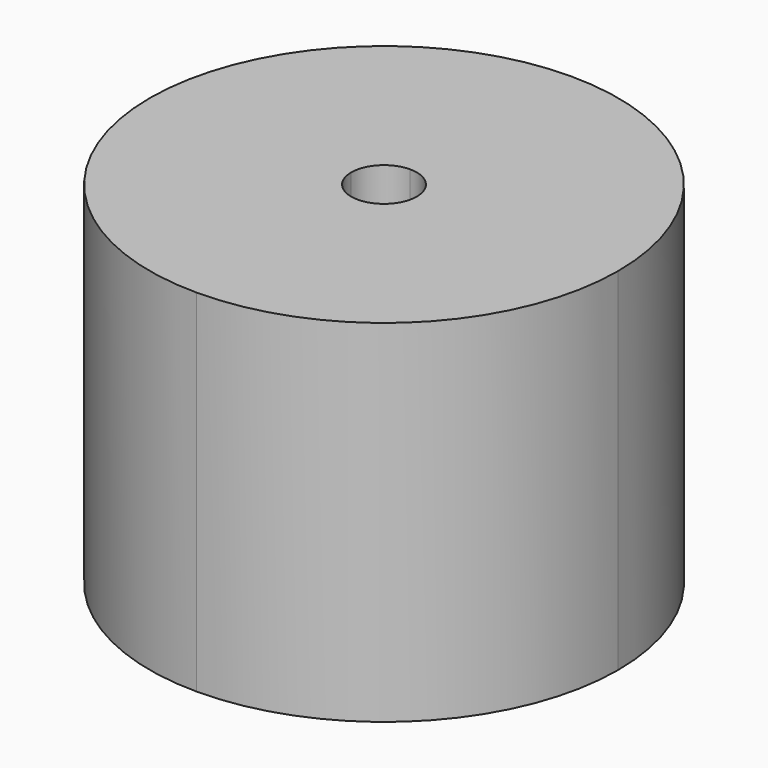
from build123d import *

# Parameters (mm, degrees)
F1_DEPTH = 19.05
F3_DEPTH = 134.874


with BuildPart() as f1:
    # F0 (on Top) → F1 (new body)
    with BuildSketch(Plane.XY):
        with BuildLine():
            Line((-12.7, 0), (0, 0))
            Line((0, 0), (0, 12.7))
            ThreePointArc((0, 12.7), (-8.9802561211, 8.9802561211), (-12.7, 0))
        make_face()
        with BuildLine():
            Line((0, 12.7), (0, 0))
            Line((0, 0), (12.7, 0))
            ThreePointArc((12.7, 0), (8.9802561211, 8.9802561211), (0, 12.7))
        make_face()
        with BuildLine():
            Line((12.7, 0), (0, 0))
            Line((0, 0), (0, -12.7))
            ThreePointArc((0, -12.7), (8.9802561211, -8.9802561211), (12.7, 0))
        make_face()
        with BuildLine():
            Line((0, -12.7), (0, 0))
            Line((0, 0), (-12.7, 0))
            ThreePointArc((-12.7, 0), (-8.9802561211, -8.9802561211), (0, -12.7))
        make_face()
    extrude(amount=F1_DEPTH)

    # F2 (on face) → F3 (cut)
    with BuildSketch(Plane.XY.offset(19.05)):
        with BuildLine():
            Line((-1.778, 0), (0, 0))
            Line((0, 0), (0, 1.778))
            ThreePointArc((0, 1.778), (-1.2572358569, 1.2572358569), (-1.778, 0))
        make_face()
        with BuildLine():
            Line((0, 1.778), (0, 0))
            Line((0, 0), (1.778, 0))
            ThreePointArc((1.778, 0), (1.2572358569, 1.2572358569), (0, 1.778))
        make_face()
        with BuildLine():
            Line((1.778, 0), (0, 0))
            Line((0, 0), (0, -1.778))
            ThreePointArc((0, -1.778), (1.2572358569, -1.2572358569), (1.778, 0))
        make_face()
        with BuildLine():
            Line((0, -1.778), (0, 0))
            Line((0, 0), (-1.778, 0))
            ThreePointArc((-1.778, 0), (-1.2572358569, -1.2572358569), (0, -1.778))
        make_face()
    extrude(amount=-F3_DEPTH, mode=Mode.SUBTRACT)


solid = f1.part
